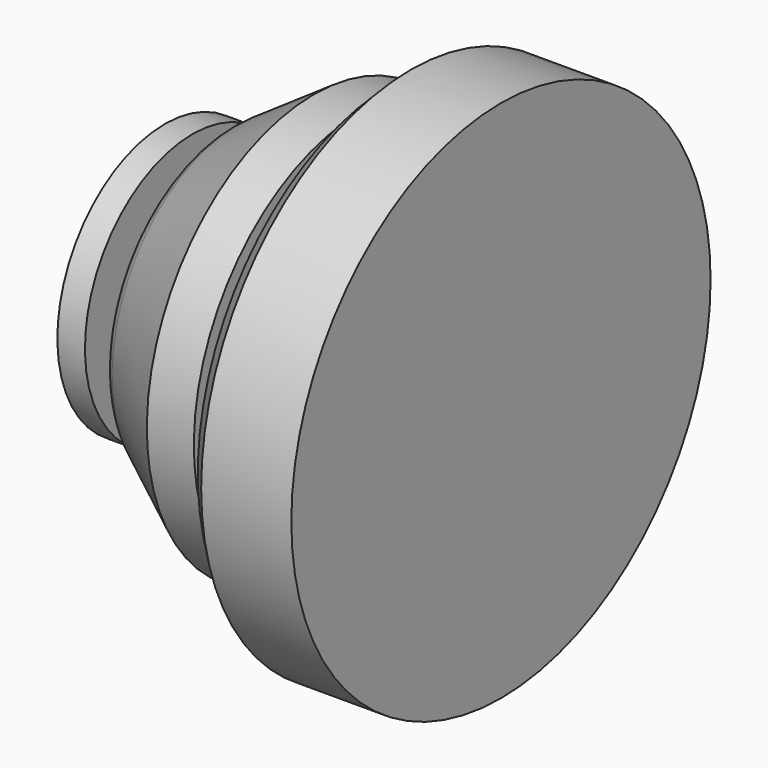
from build123d import *

# Parameters (mm, degrees)
F2_R    = 10.6144552681
F3_SIZE = 5


# Not quite as in the source:
# - a feature of the source that left no trace in its solid (it failed there, or was rolled back) is left out


with BuildPart() as f1:
    # F0 (on Front) → F1 (revolve)
    with BuildSketch(Plane.XZ):
        Polygon((-98.2463732362, 0), (0, 0), (0, 76.5963345766), (-31.3552282751, 76.5963345766), (-31.3552282751, 47.6300790906), (-40.9111082554, 47.6300790906), (-40.9111082554, 61.0680393875), (-54.6476840973, 61.0680393875), (-81.5235897899, 42.8521446884), (-81.5235897899, 20.1569329947), (-90.1836082339, 20.1569329947), (-90.1836082339, 39.2686873674), (-98.2463732362, 39.2686873674), align=None)
    revolve(axis=Axis((-49.1231866181, 0, 0), (-1, 0, 0)))

    # F2
    f2_edges = [f1.edges().sort_by_distance(p)[0] for p in [
        (-81.52359, 0, -42.852145),
    ]]
    fillet(f2_edges, radius=F2_R)

    # F3
    f3_edges = [f1.edges().sort_by_distance(p)[0] for p in [
        (-31.355228, 0, -76.596335),
    ]]
    chamfer(f3_edges, length=F3_SIZE)


solid = f1.part
